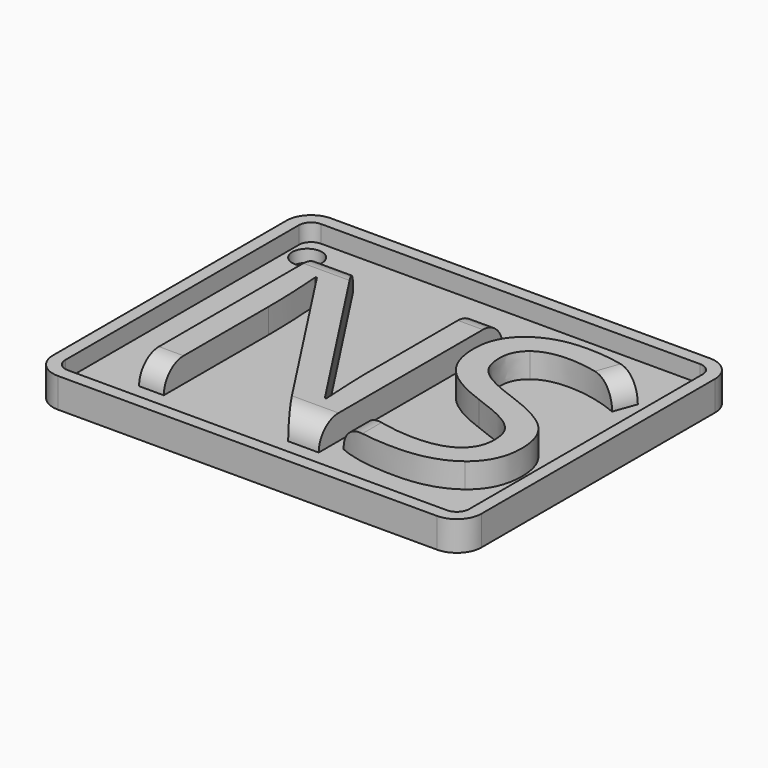
from build123d import *

# Parameters (mm, degrees)
F0_W         = 86.5714140236
F0_H         = 68.943746388
F1_DEPTH     = 6
F2_W         = 79.0391676128
F2_H         = 60.1468821988
F3_DEPTH     = 6
F4_R         = 5
F5_T         = -2.5
F7_DEPTH     = 5
F8_TEXT_SIZE = 65.0627318666
F9_DEPTH     = 5
F11_D        = 6
F12_R        = 4.99999
F13_R        = 4.99999
F14_R        = 4.99999


# Not quite as in the source:
# - a fillet or chamfer is up to 0.001 mm smaller than in the source, because OpenCascade refuses the exact size
# - Text() gives the source's letters only with a copy of the font that has no kerning and outlines rounded to 1/6400 em; it was checked with that copy


with BuildPart() as f1:
    # F0 (on Top) → F1 (new body)
    with BuildSketch(Plane.XY):
        with Locations((3.5255346447, 15.9628279507)):
            Rectangle(F0_W, F0_H)
    extrude(amount=F1_DEPTH)

    # F2 (on face) → F3 (join)
    with BuildSketch(Plane.XY.offset(6)):
        with Locations((3.0844528228, 16.0970021971)):
            Rectangle(F2_W, F2_H)
    extrude(amount=-F3_DEPTH)

    # F4
    f4_edges = [f1.edges().sort_by_distance(p)[0] for p in [
        (-39.760172, -18.509045, 3),
        (46.811242, -18.509045, 3),
        (-39.760172, 50.434701, 3),
        (46.811242, 50.434701, 3),
    ]]
    fillet(f4_edges, radius=F4_R)

    # F5
    f5_openings = [f1.faces().sort_by_distance(p)[0] for p in [
        (3.525535, 15.962828, 6),
    ]]
    offset(amount=F5_T, openings=f5_openings)

    # F6 (on face) → F7 (join)
    with BuildSketch(Plane.XY.offset(2.5)):
        with BuildLine():
            add(Edge.make_bspline(
                [(39.6344235432, 5.6789298154), (39.6344235432, -0.1484769715), (35.4064128148, -3.4149172601)],
                knots=[0, 0, 0, 1, 1, 1], degree=2))
            add(Edge.make_bspline(
                [(37.0251369222, 13.0429165013), (39.6344235432, 10.2016932918), (39.6344235432, 5.6789298154)],
                knots=[0, 0, 0, 1, 1, 1], degree=2))
            add(Edge.make_bspline(
                [(27.4674166697, 18.3581299886), (34.4158503012, 15.8841397109), (37.0251369222, 13.0429165013)],
                knots=[0, 0, 0, 1, 1, 1], degree=2))
            add(Edge.make_bspline(
                [(21.3210970736, 21.0592248426), (23.3312141742, 19.8367257405), (27.4674166697, 18.3581299886)],
                knots=[0, 0, 0, 1, 1, 1], degree=2))
            add(Edge.make_bspline(
                [(18.4653778272, 23.750655672), (19.3109799729, 22.2817239446), (21.3210970736, 21.0592248426)],
                knots=[0, 0, 0, 1, 1, 1], degree=2))
            add(Edge.make_bspline(
                [(17.6197756815, 27.5099612112), (17.6197756815, 25.2195873994), (18.4653778272, 23.750655672)],
                knots=[0, 0, 0, 1, 1, 1], degree=2))
            add(Edge.make_bspline(
                [(19.9149815056, 32.3709655459), (17.6197756815, 30.6217771073), (17.6197756815, 27.5099612112)],
                knots=[0, 0, 0, 1, 1, 1], degree=2))
            add(Edge.make_bspline(
                [(26.288405678, 34.1201539844), (22.2101873296, 34.1201539844), (19.9149815056, 32.3709655459)],
                knots=[0, 0, 0, 1, 1, 1], degree=2))
            add(Edge.make_bspline(
                [(36.9188326525, 31.8297801726), (31.4489947729, 34.1201539844), (26.288405678, 34.1201539844)],
                knots=[0, 0, 0, 1, 1, 1], degree=2))
            Line((36.9188326525, 31.8297801726), (38.5230607232, 36.2945595019))
            add(Edge.make_bspline(
                [(26.4140379968, 38.7105656325), (32.9952386965, 38.7105656325), (38.5230607232, 36.2945595019)],
                knots=[0, 0, 0, 1, 1, 1], degree=2))
            add(Edge.make_bspline(
                [(16.2619802362, 35.6905579692), (20.0937659592, 38.7105656325), (26.4140379968, 38.7105656325)],
                knots=[0, 0, 0, 1, 1, 1], degree=2))
            add(Edge.make_bspline(
                [(12.4301945131, 27.5679453583), (12.4301945131, 32.670550306), (16.2619802362, 35.6905579692)],
                knots=[0, 0, 0, 1, 1, 1], degree=2))
            add(Edge.make_bspline(
                [(15.0733052199, 19.6869333604), (12.4301945131, 22.7069410236), (12.4301945131, 27.5679453583)],
                knots=[0, 0, 0, 1, 1, 1], degree=2))
            add(Edge.make_bspline(
                [(23.8723995474, 14.4635281061), (17.7164159268, 16.6669256972), (15.0733052199, 19.6869333604)],
                knots=[0, 0, 0, 1, 1, 1], degree=2))
            add(Edge.make_bspline(
                [(30.4391042103, 11.6561289824), (28.2791947296, 12.8979561335), (23.8723995474, 14.4635281061)],
                knots=[0, 0, 0, 1, 1, 1], degree=2))
            add(Edge.make_bspline(
                [(33.5219280329, 8.9502021162), (32.599013691, 10.4143018313), (30.4391042103, 11.6561289824)],
                knots=[0, 0, 0, 1, 1, 1], degree=2))
            add(Edge.make_bspline(
                [(34.4448423748, 5.1957285893), (34.4448423748, 7.486102401), (33.5219280329, 8.9502021162)],
                knots=[0, 0, 0, 1, 1, 1], degree=2))
            add(Edge.make_bspline(
                [(31.8452197783, -0.23062118), (34.4448423748, 1.7166797613), (34.4448423748, 5.1957285893)],
                knots=[0, 0, 0, 1, 1, 1], degree=2))
            add(Edge.make_bspline(
                [(24.1140001605, -2.1779221212), (29.2455971818, -2.1779221212), (31.8452197783, -0.23062118)],
                knots=[0, 0, 0, 1, 1, 1], degree=2))
            add(Edge.make_bspline(
                [(17.7744000739, -1.5111044292), (20.9731921908, -2.1779221212), (24.1140001605, -2.1779221212)],
                knots=[0, 0, 0, 1, 1, 1], degree=2))
            add(Edge.make_bspline(
                [(11.8503530418, 0.2960681565), (14.575607957, -0.8442867371), (17.7744000739, -1.5111044292)],
                knots=[0, 0, 0, 1, 1, 1], degree=2))
            Line((11.8503530418, 0.2960681565), (11.8503530418, -4.6519123989))
            add(Edge.make_bspline(
                [(23.9303836946, -6.6813575486), (16.0831957825, -6.6813575486), (11.8503530418, -4.6519123989)],
                knots=[0, 0, 0, 1, 1, 1], degree=2))
            add(Edge.make_bspline(
                [(35.4064128148, -3.4149172601), (31.1784020863, -6.6813575486), (23.9303836946, -6.6813575486)],
                knots=[0, 0, 0, 1, 1, 1], degree=2))
        make_face()
    extrude(amount=F7_DEPTH)

    # F8 (on face) → F9 (join)
    with BuildSketch(Plane.XY.offset(2.5)):
        with Locations((-33.1578962505, -8.0003058538)):
            Text('N', F8_TEXT_SIZE, font='Open Sans', text_align=(TextAlign.LEFT, TextAlign.BOTTOM))
    extrude(amount=F9_DEPTH)

    # F11 (through all)
    with Locations(Plane.XY.offset(2.5)):
        with Locations((-33.5434526205, 42.8932085633)):
            Hole(F11_D / 2)

    # F12 (radius 5 in the source; OpenCascade refuses exactly that, so slightly less here)
    f12_edges = [f1.edges().sort_by_distance(p)[0] for p in [
        (11.850353, -2.177922, 7.5),
    ]]
    fillet(f12_edges, radius=F12_R)

    # F13 (radius 5 in the source; OpenCascade refuses exactly that, so slightly less here)
    f13_edges = [f1.edges().sort_by_distance(p)[0] for p in [
        (37.720947, 34.06217, 7.5),
    ]]
    fillet(f13_edges, radius=F13_R)

    # F14 (radius 5 in the source; OpenCascade refuses exactly that, so slightly less here)
    f14_edges = [f1.edges().sort_by_distance(p)[0] for p in [
        (6.42871, -8.000306, 7.5),
        (-24.27785, -8.000306, 7.5),
        (6.982759, 38.448385, 7.5),
        (-23.7238, 38.448385, 7.5),
    ]]
    fillet(f14_edges, radius=F14_R)


solid = f1.part
